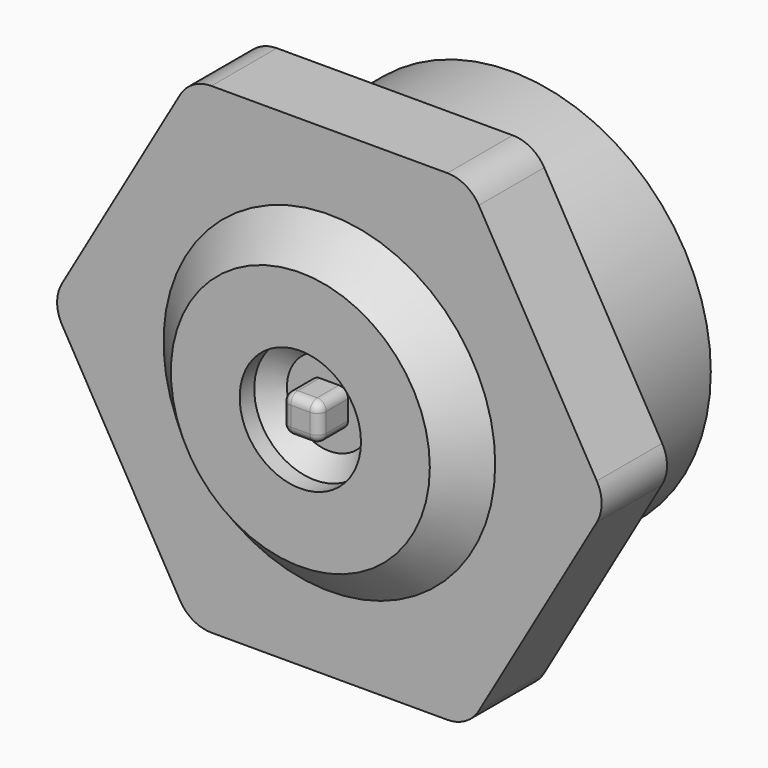
from build123d import *

# Parameters (mm, degrees)
F0_R     = 11
F1_DEPTH = 8
F3_DEPTH = 4.5
F4_R     = 12.1301412178
F4_R_2   = 3.338839996
F5_DEPTH = 2
F7_SIZE  = 1
F8_W     = 2.0535623771
F8_H     = 2.0535623771
F9_DEPTH = 2
F10_R    = 0.5


# Not quite as in the source:
# - a fillet or chamfer that OpenCascade refuses, or shapes differently, is made with other operations: its cross-section is extruded or revolved along the edge and cut away or added


with BuildPart() as f1:
    # F0 (on Front) → F1 (new body)
    with BuildSketch(Plane.XZ):
        Circle(F0_R)
    extrude(amount=F1_DEPTH)

    # F2 (on face) → F3 (join)
    with BuildSketch(Plane.XZ.offset(8)):
        with BuildLine():
            Line((6.4951905284, 13.25), (-6.4951905284, 13.25))
            ThreePointArc((-6.4951905284, 13.25), (-7.4951905284, 12.9820508076), (-8.227241336, 12.25))
            Line((-8.227241336, 12.25), (-14.7224318643, 1))
            ThreePointArc((-14.7224318643, 1), (-14.9903810568, 0), (-14.7224318643, -1))
            Line((-14.7224318643, -1), (-8.227241336, -12.25))
            ThreePointArc((-8.227241336, -12.25), (-7.4951905284, -12.9820508076), (-6.4951905284, -13.25))
            Line((-6.4951905284, -13.25), (6.4951905284, -13.25))
            ThreePointArc((6.4951905284, -13.25), (7.4951905284, -12.9820508076), (8.227241336, -12.25))
            Line((8.227241336, -12.25), (14.7224318643, -1))
            ThreePointArc((14.7224318643, -1), (14.9903810568, 0), (14.7224318643, 1))
            Line((14.7224318643, 1), (8.227241336, 12.25))
            ThreePointArc((8.227241336, 12.25), (7.4951905284, 12.9820508076), (6.4951905284, 13.25))
        make_face()
    extrude(amount=F3_DEPTH)

    # F4 (on face) → F5 (join)
    with BuildSketch(Plane.XZ.offset(12.5)):
        Circle(F4_R)
        Circle(F4_R_2, mode=Mode.SUBTRACT)
    extrude(amount=F5_DEPTH)

    # F6: chamfer of 5 on 1 edges, made by hand


with BuildPart() as f6_tool2:
    # F6_s3 → F6_t4 (revolve)
    with BuildSketch(Plane.XY):
        Polygon((12.1301412178, -9.5), (7.1301412178, -14.5), (12.1301412178, -14.5), align=None)
    revolve(axis=Axis((0, -14.5, 0), (0, -1, 0)))

    split(bisect_by=Plane.XZ.offset(12.5), keep=Keep.TOP)


with BuildPart() as f1_1:
    add(f1.part)

    # F6_t1: cut F6_tool2
    add(f6_tool2.part, mode=Mode.SUBTRACT)

    # F7
    f7_edges = [f1_1.edges().sort_by_distance(p)[0] for p in [
        (-3.33884, -12.5, 0),
    ]]
    chamfer(f7_edges, length=F7_SIZE)

    # F8 (on face) → F9 (join)
    with BuildSketch(Plane.XZ.offset(12.5)):
        Rectangle(F8_W, F8_H)
    extrude(amount=F9_DEPTH)

    # F10
    f10_edges = [f1_1.edges().sort_by_distance(p)[0] for p in [
        (1.026781, -13.5, -1.026781),
        (-1.026781, -13.5, -1.026781),
        (-1.026781, -13.5, 1.026781),
        (1.026781, -13.5, 1.026781),
        (1.026781, -14.5, 0),
        (0, -14.5, 1.026781),
        (-1.026781, -14.5, 0),
        (0, -14.5, -1.026781),
    ]]
    fillet(f10_edges, radius=F10_R)


solid = f1_1.part
